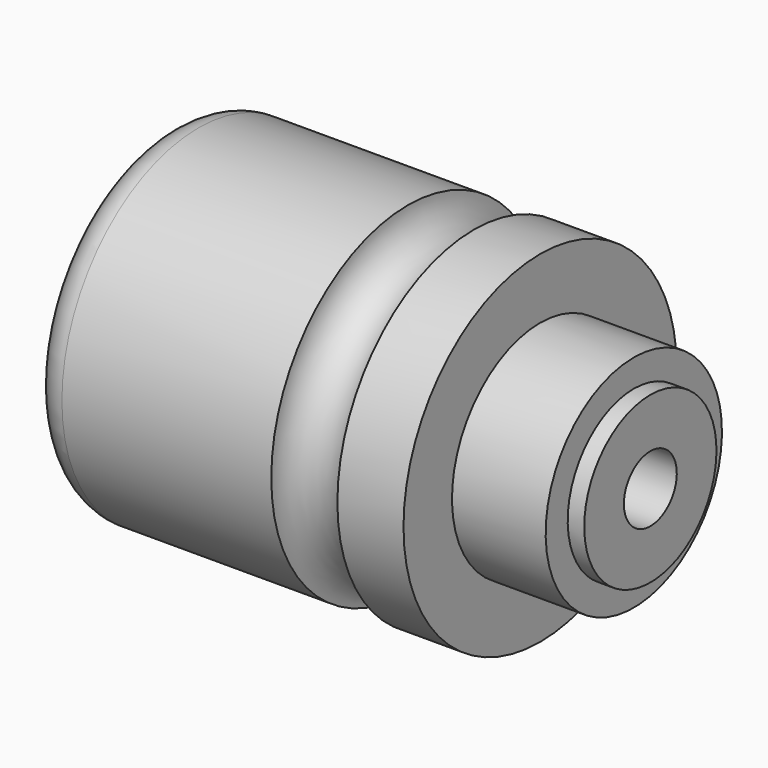
from build123d import *

# Parameters (mm, degrees)
F4_R = 5.99999


# Not quite as in the source:
# - a fillet or chamfer is up to 0.001 mm smaller than in the source, because OpenCascade refuses the exact size


with BuildPart() as f1:
    # F0 (on Front) → F1 (revolve)
    with BuildSketch(Plane.XZ):
        with BuildLine():
            Line((0, 31), (0, 0))
            Line((0, 0), (88, 0))
            Line((88, 0), (88, 15))
            Line((88, 15), (85, 15))
            Line((85, 15), (85, 20))
            Line((85, 20), (68, 20))
            Line((68, 20), (68, 31))
            Line((68, 31), (56, 31))
            ThreePointArc((56, 31), (50, 25), (44, 31))
            Line((44, 31), (0, 31))
        make_face()
    revolve(axis=Axis((45.4589584282, 0, 0), (1, 0, 0)))

    # F2 (on Front) → F3 (revolve, cut)
    with BuildSketch(Plane.XZ):
        Polygon((0, 25), (0, 0), (88, 0), (88, 6), (30, 6), (30, 16), (22, 16), (22, 20.5), (19, 20.5), (19, 12.5), (12, 12.5), (12, 16), (1.5, 16), (1.5, 25), align=None)
    revolve(axis=Axis((-7.9182099137, 0, 0), (-1, 0, 0)), mode=Mode.SUBTRACT)

    # F4 (radius 6 in the source; OpenCascade refuses exactly that, so slightly less here)
    f4_edges = [f1.edges().sort_by_distance(p)[0] for p in [
        (0, 0, -31),
    ]]
    fillet(f4_edges, radius=F4_R)


solid = f1.part
